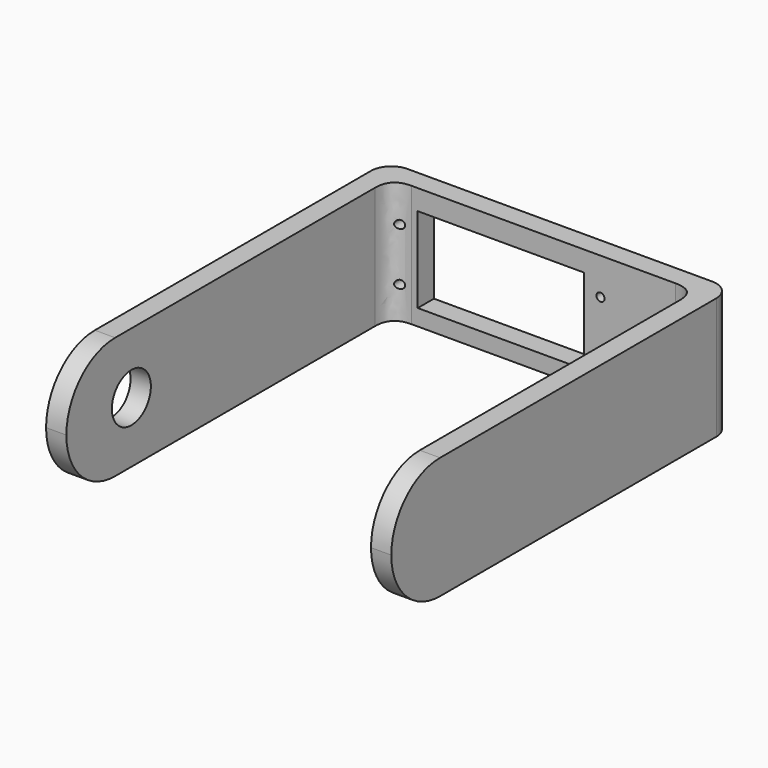
from build123d import *

# Parameters (mm, degrees)
F1_DEPTH    = 30
F3_START    = 37.5
F2_R        = 3.5
F3_DEPTH    = 2.5
F5_START    = -37.5
F4_R        = 6
F5_DEPTH    = 5
F6_R        = 14.99999
F7_R        = 5
F8_T1_DEPTH = 30
F10_START   = -33
F9_W        = 41
F9_H        = 21
F10_DEPTH   = 12
F12_START   = -35
F11_R       = 1
F12_DEPTH   = 10


# Not quite as in the source:
# - a fillet or chamfer that OpenCascade refuses, or shapes differently, is made with other operations: its cross-section is extruded or revolved along the edge and cut away or added
# - a fillet or chamfer is up to 0.001 mm smaller than in the source, because OpenCascade refuses the exact size


with BuildPart() as f1:
    # F0 (on Top) → F1 (new body)
    with BuildSketch(Plane.XY):
        Polygon((-42.5, -62.7966840421), (-37.5, -62.7966840421), (-37.5, 37.2033159579), (37.5, 37.2033159579), (37.5, -62.7966840421), (42.5, -62.7966840421), (42.5, 42.2033159579), (-42.5, 42.2033159579), align=None)
    extrude(amount=F1_DEPTH)

    # F2 (on Right) → F3 (cut)
    with BuildSketch(Plane.YZ.offset(F3_START)):
        with Locations((-42.7966840421, 15)):
            Circle(F2_R)
    extrude(amount=F3_DEPTH, mode=Mode.SUBTRACT)

    # F4 (on Right) → F5 (cut)
    with BuildSketch(Plane.YZ.offset(F5_START)):
        with Locations((-42.7966840421, 15)):
            Circle(F4_R)
    extrude(amount=-F5_DEPTH, mode=Mode.SUBTRACT)

    # F6 (radius 15 in the source; OpenCascade refuses exactly that, so slightly less here)
    f6_edges = [f1.edges().sort_by_distance(p)[0] for p in [
        (40, -62.796684, 30),
        (40, -62.796684, 0),
        (-40, -62.796684, 30),
        (-40, -62.796684, 0),
    ]]
    fillet(f6_edges, radius=F6_R)

    # F7
    f7_edges = [f1.edges().sort_by_distance(p)[0] for p in [
        (-42.5, 42.203316, 15),
        (42.5, 42.203316, 15),
    ]]
    fillet(f7_edges, radius=F7_R)

    # F8: fillet of radius 5 on 2 edges, made by hand

    # F8_s2 → F8_t1 (join)
    with BuildSketch(Plane.XY):
        with BuildLine():
            add(Edge.make_bspline(
                [(-37.5, 32.2033159579), (-37.5, 37.2033159579), (-32.5, 37.2033159579)],
                knots=[0, 0, 0, 1, 1, 1], degree=2, weights=[1, 1, 1]))
            Line((-32.5, 37.2033159579), (-37.5, 37.2033159579))
            Line((-37.5, 37.2033159579), (-37.5, 32.2033159579))
        make_face()
        with BuildLine():
            add(Edge.make_bspline(
                [(32.5, 37.2033159579), (37.5, 37.2033159579), (37.5, 32.2033159579)],
                knots=[0, 0, 0, 1, 1, 1], degree=2, weights=[1, 1, 1]))
            Line((37.5, 32.2033159579), (37.5, 37.2033159579))
            Line((37.5, 37.2033159579), (32.5, 37.2033159579))
        make_face()
    extrude(amount=F8_T1_DEPTH)

    # F9 (on Front) → F10 (cut)
    with BuildSketch(Plane.XZ.offset(F10_START)):
        with Locations((-10.5, 14.5)):
            Rectangle(F9_W, F9_H)
    extrude(amount=-F10_DEPTH, mode=Mode.SUBTRACT)

    # F11 (on Front) → F12 (cut)
    with BuildSketch(Plane.XZ.offset(F12_START)):
        with Locations((14, 21)):
            Circle(F11_R)
        with Locations((14, 8)):
            Circle(F11_R)
        with Locations((-35, 21)):
            Circle(F11_R)
        with Locations((-35, 8)):
            Circle(F11_R)
    extrude(amount=-F12_DEPTH, mode=Mode.SUBTRACT)


solid = f1.part
